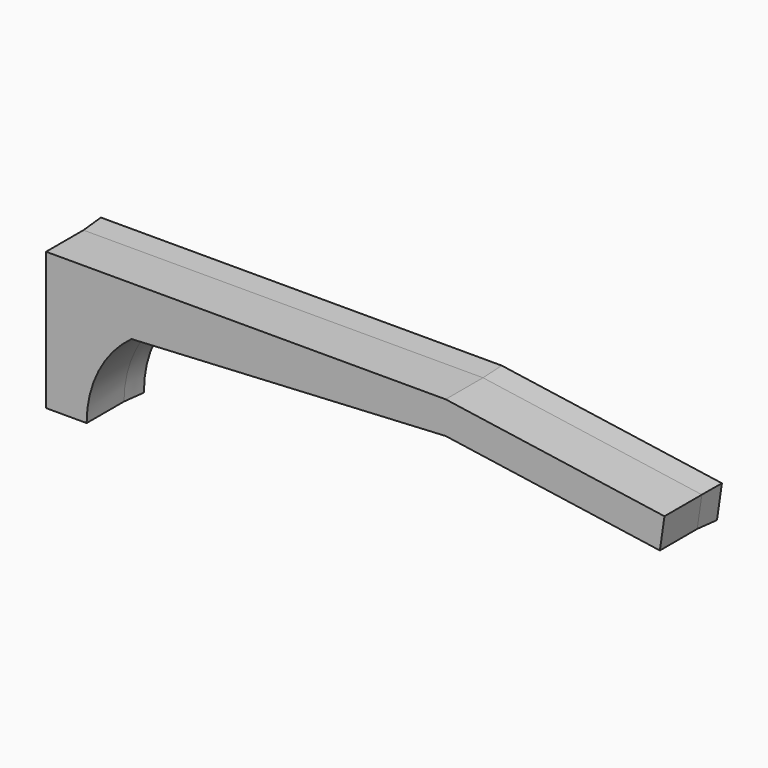
from build123d import *

# Parameters (mm, degrees)
F1_DEPTH               = 19
F2_DEPTH               = 19
DRAFT_F2_DRAFTED_ANGLE = -3
F3_DEPTH               = 19


# Not quite as in the source:
# - an extrude with a draft is written as a straight extrude whose walls are then drafted


with BuildPart() as f1:
    # F0 (on Front) → F1 (new body)
    with BuildSketch(Plane.XZ):
        with BuildLine():
            Line((220.2389582992, 36.7874841094), (-104.7610417008, 36.7874841094))
            Line((-104.7610417008, 36.7874841094), (-104.7610417008, -75.2125158906))
            Line((-104.7610417008, -75.2125158906), (-71.7610417008, -75.2125158906))
            ThreePointArc((-71.7610417008, -75.2125158906), (-62.1278945979, -34.825302405), (-35.3026326909, -3.1341386546))
            Line((-35.3026326909, -3.1341386546), (220.2389582992, 10.5146205185))
            Line((220.2389582992, 10.5146205185), (394.501495504, -14.7982633169))
            Line((394.501495504, -14.7982633169), (398.2389582992, 10.9317069873))
            Line((398.2389582992, 10.9317069873), (220.2389582992, 36.7874841094))
        make_face()
    extrude(amount=F1_DEPTH)


with BuildPart() as f2_drafted:
    # F0 (on Front) → F2 (new body)
    with BuildSketch(Plane.XZ):
        with BuildLine():
            Line((220.2389582992, 36.7874841094), (-104.7610417008, 36.7874841094))
            Line((-104.7610417008, 36.7874841094), (-104.7610417008, -75.2125158906))
            Line((-104.7610417008, -75.2125158906), (-71.7610417008, -75.2125158906))
            ThreePointArc((-71.7610417008, -75.2125158906), (-62.1278945979, -34.825302405), (-35.3026326909, -3.1341386546))
            Line((-35.3026326909, -3.1341386546), (220.2389582992, 10.5146205185))
            Line((220.2389582992, 10.5146205185), (394.501495504, -14.7982633169))
            Line((394.501495504, -14.7982633169), (398.2389582992, 10.9317069873))
            Line((398.2389582992, 10.9317069873), (220.2389582992, 36.7874841094))
        make_face()
    extrude(amount=-F2_DEPTH)

    # draft_F2_drafted
    draft_f2_drafted_walls = [f2_drafted.faces().sort_by_distance(p)[0] for p in [
        (309.2389582992, 12.6666666667, 23.8595955484),
        (57.7389582992, 12.6666666667, 36.7874841094),
        (-104.7610417008, 12.6666666667, -19.2125158906),
        (-88.2610417008, 12.6666666667, -75.2125158906),
        (-62.1278945979, 12.6666666667, -34.825302405),
        (92.4681628041, 12.6666666667, 3.690240932),
        (307.3702269016, 12.6666666667, -2.1418213992),
        (396.3702269016, 12.6666666667, -1.9332781648),
    ]]
    draft(draft_f2_drafted_walls, neutral_plane=Plane(origin=(0, 0, 0), x_dir=(1, 0, 0), z_dir=(0, 1, 0)), angle=DRAFT_F2_DRAFTED_ANGLE)


with BuildPart() as f1_1:
    add(f1.part)

    # join_F2_drafted: union F2_drafted
    add(f2_drafted.part)

    # F3 (add): a face of the model
    f3_faces = [f1_1.faces().sort_by_distance(p)[0] for p in [
        (88.4015845817, -19, 8.2561337658),
    ]]
    extrude(f3_faces, amount=F3_DEPTH)


solid = f1_1.part
